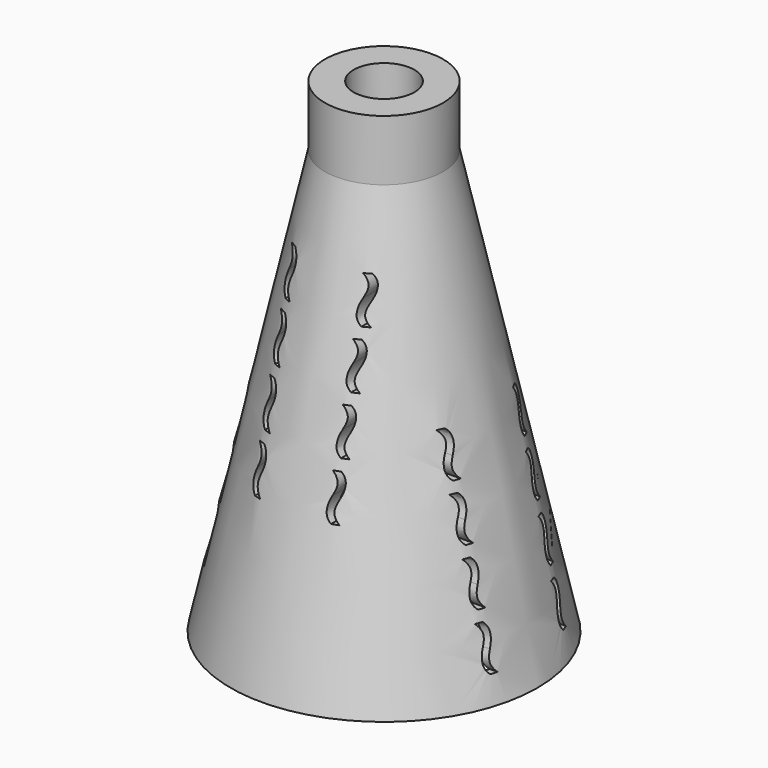
from build123d import *

# Parameters (mm, degrees)
F0_W         = 4.7292866558
F0_H         = 9.9851343036
F3_TEXT_SIZE = 14.8629215786
F4_DEPTH     = 65.2607893305
F6_TEXT_SIZE = 14.8629215786
F7_DEPTH     = 50.2607894305


# Not quite as in the source:
# - Text() gives the source's letters only with a copy of the font that has no kerning and outlines rounded to 1/6400 em; it was checked with that copy


with BuildPart() as f1:
    # F0 (on Front) → F1 (revolve)
    with BuildSketch(Plane.XZ):
        Polygon((9.7292866558, 70), (5, 70), (24.2957451861, 0), (25.2597893305, 0.2657421451), align=None)
        with Locations((7.3646433279, 74.9925671518)):
            Rectangle(F0_W, F0_H)
    revolve(axis=Axis((0, 0, 35), (0, 0, 1)))

    # F3 (on offset) → F4 (cut, through all)
    with BuildSketch(Plane.XZ.offset(40)):
        with Locations(Location((1.1000001105, 50.5156947731), (0, 0, -90))):
            Text('~', F3_TEXT_SIZE, font='Open Sans', text_align=(TextAlign.LEFT, TextAlign.BOTTOM))
        with Locations(Location((1.1000001105, 41.8232079811), (0, 0, -90))):
            Text('~', F3_TEXT_SIZE, font='Open Sans', text_align=(TextAlign.LEFT, TextAlign.BOTTOM))
        with Locations(Location((1.1000001105, 33.1307208381), (0, 0, -90))):
            Text('~', F3_TEXT_SIZE, font='Open Sans', text_align=(TextAlign.LEFT, TextAlign.BOTTOM))
        with Locations(Location((1.1000001105, 59.1763776011), (0, 0, -90))):
            Text('~', F3_TEXT_SIZE, font='Open Sans', text_align=(TextAlign.LEFT, TextAlign.BOTTOM))
        with Locations(Location((13.0563051207, 112.1757461189), (0, 0, -90))):
            Text('~', F3_TEXT_SIZE, font='Open Sans', text_align=(TextAlign.LEFT, TextAlign.BOTTOM))
        with Locations(Location((13.0563051207, 103.4832593269), (0, 0, -90))):
            Text('~', F3_TEXT_SIZE, font='Open Sans', text_align=(TextAlign.LEFT, TextAlign.BOTTOM))
        with Locations(Location((13.0563051207, 94.7907721839), (0, 0, -90))):
            Text('~', F3_TEXT_SIZE, font='Open Sans', text_align=(TextAlign.LEFT, TextAlign.BOTTOM))
        with Locations(Location((13.0563051207, 120.8364289469), (0, 0, -90))):
            Text('~', F3_TEXT_SIZE, font='Open Sans', text_align=(TextAlign.LEFT, TextAlign.BOTTOM))
        with Locations(Location((-11.429881677, 50.5220910965), (0, 0, -90))):
            Text('~', F3_TEXT_SIZE, font='Open Sans', text_align=(TextAlign.LEFT, TextAlign.BOTTOM))
        with Locations(Location((-11.429881677, 41.8296043045), (0, 0, -90))):
            Text('~', F3_TEXT_SIZE, font='Open Sans', text_align=(TextAlign.LEFT, TextAlign.BOTTOM))
        with Locations(Location((-11.429881677, 33.1371171615), (0, 0, -90))):
            Text('~', F3_TEXT_SIZE, font='Open Sans', text_align=(TextAlign.LEFT, TextAlign.BOTTOM))
        with Locations(Location((-11.429881677, 59.1827739245), (0, 0, -90))):
            Text('~', F3_TEXT_SIZE, font='Open Sans', text_align=(TextAlign.LEFT, TextAlign.BOTTOM))
    extrude(amount=-F4_DEPTH, mode=Mode.SUBTRACT)

    # F6 (on offset) → F7 (cut, through all)
    with BuildSketch(Plane.YZ.offset(25)):
        with Locations(Location((-12.2548127547, 29.60386383), (0, 0, -90))):
            Text('~', F6_TEXT_SIZE, font='Open Sans', text_align=(TextAlign.LEFT, TextAlign.BOTTOM))
        with Locations(Location((-12.2548127547, 20.911377038), (0, 0, -90))):
            Text('~', F6_TEXT_SIZE, font='Open Sans', text_align=(TextAlign.LEFT, TextAlign.BOTTOM))
        with Locations(Location((-12.2548127547, 12.218889895), (0, 0, -90))):
            Text('~', F6_TEXT_SIZE, font='Open Sans', text_align=(TextAlign.LEFT, TextAlign.BOTTOM))
        with Locations(Location((-12.2548127547, 38.264546658), (0, 0, -90))):
            Text('~', F6_TEXT_SIZE, font='Open Sans', text_align=(TextAlign.LEFT, TextAlign.BOTTOM))
        with Locations(Location((3.200000152, 29.60386383), (0, 0, -90))):
            Text('~', F6_TEXT_SIZE, font='Open Sans', text_align=(TextAlign.LEFT, TextAlign.BOTTOM))
        with Locations(Location((3.200000152, 20.911377038), (0, 0, -90))):
            Text('~', F6_TEXT_SIZE, font='Open Sans', text_align=(TextAlign.LEFT, TextAlign.BOTTOM))
        with Locations(Location((3.200000152, 12.218889895), (0, 0, -90))):
            Text('~', F6_TEXT_SIZE, font='Open Sans', text_align=(TextAlign.LEFT, TextAlign.BOTTOM))
        with Locations(Location((3.200000152, 38.264546658), (0, 0, -90))):
            Text('~', F6_TEXT_SIZE, font='Open Sans', text_align=(TextAlign.LEFT, TextAlign.BOTTOM))
    extrude(amount=-F7_DEPTH, mode=Mode.SUBTRACT)


solid = f1.part
